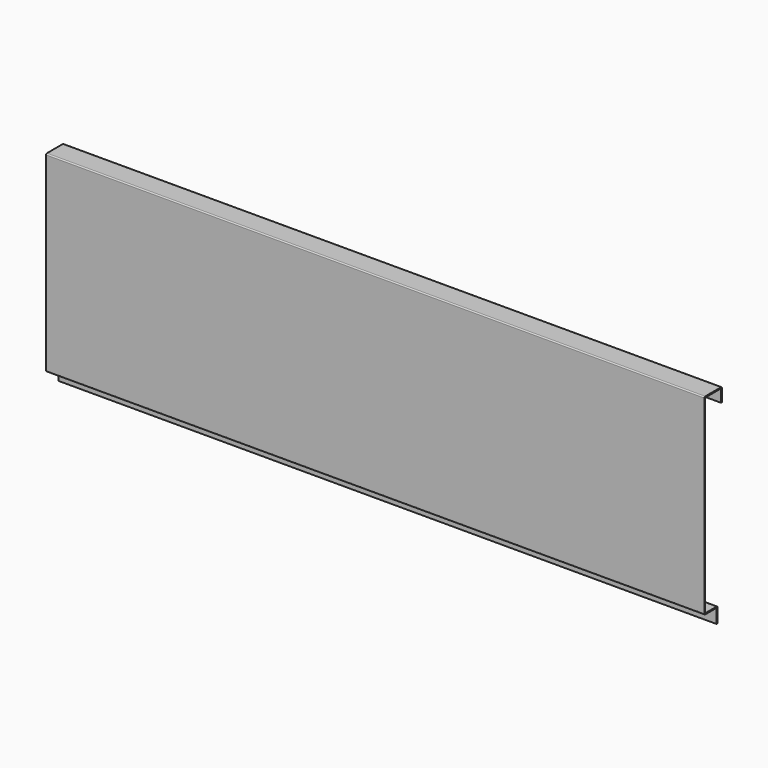
from build123d import *

# Parameters (mm, degrees)
F1_DEPTH = 1200
F2_R     = 2


# Not quite as in the source:
# - a feature names something its author has since deleted; it is built from what else it names


with BuildPart() as f1:
    # F0 (on Right) → F1 (new body)
    with BuildSketch(Plane.YZ):
        Polygon((-19.8378913403, 427.8021101952), (-19.8378913403, 404.8021101952), (-17.8378913403, 404.8021101952), (-17.8378913403, 429.8021101952), (-57.8378913403, 429.8021101952), (-57.8378913403, 79.8021101952), (-29.8378913403, 79.8021101952), (-29.8378913403, 53.8021101952), (-27.8378913403, 53.8021101952), (-27.8378913403, 81.8021101952), (-55.8378913403, 81.8021101952), (-55.8378913403, 427.8021101952), align=None)
    extrude(amount=F1_DEPTH)

    # F2
    f2_edges = [f1.edges().sort_by_distance(p)[0] for p in [
        (600, -57.837891, 429.80211),
        (600, -17.837891, 429.80211),
        (600, -57.837891, 79.80211),
        (600, -27.837891, 81.80211),
        (600, -55.837891, 81.80211),
        (600, -29.837891, 79.80211),
        (600, -19.837891, 427.80211),
        (600, -55.837891, 427.80211),
    ]]
    fillet(f2_edges, radius=F2_R)


solid = f1.part
